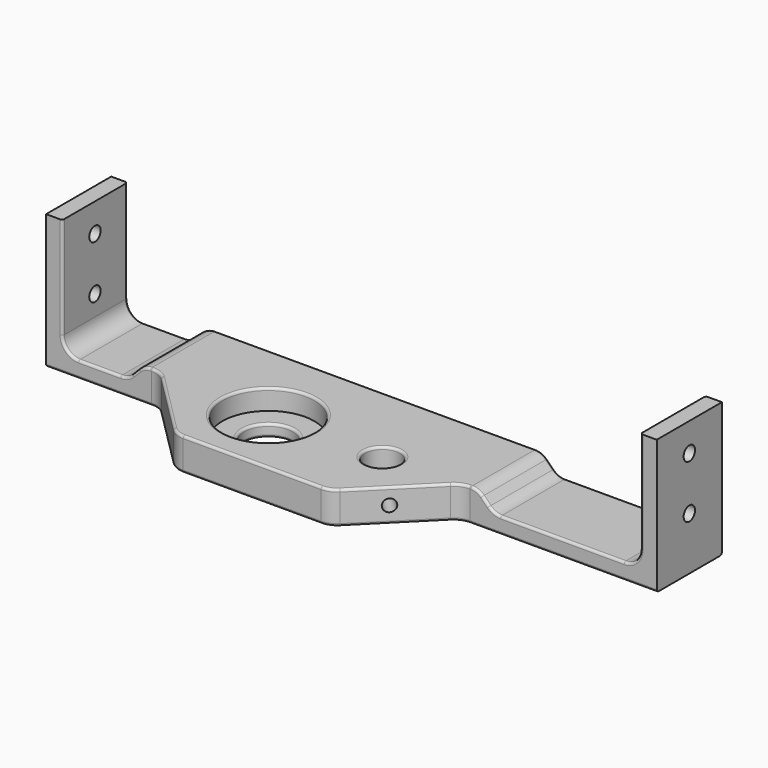
from build123d import *

# Parameters (mm, degrees)
F0_R      = 11.3
F0_R_2    = 4.3
F1_DEPTH  = 8
F0_R_3    = 6
F2_DEPTH  = 3
F4_W      = 4
F4_H      = 20
F5_DEPTH  = 25
F7_DEPTH  = 25
F8_R      = 0.6
F9_R      = 5
F10_R     = 4
F11_R     = 1.75
F12_DEPTH = 150.001
F13_R     = 0.6
F14_R     = 1.5
F15_DEPTH = 15


with BuildPart() as f1:
    # F0 (on Top) → F1 (new body)
    with BuildSketch(Plane.XY):
        Polygon((72.1656017255, 12.1974679563), (-77.8343982745, 12.1974679563), (-77.8343982745, -7.8025320437), (-49.8343982745, -7.8025320437), (-31.8343982745, -25.8025320437), (6.1656017255, -25.8025320437), (24.1656017255, -7.8025320437), (72.1656017255, -7.8025320437), align=None)
        with Locations((-22.4343982745, -8.8025320437)):
            Circle(F0_R, mode=Mode.SUBTRACT)
        with Locations((5.5656017255, -8.8025320437)):
            Circle(F0_R_2, mode=Mode.SUBTRACT)
    extrude(amount=F1_DEPTH)

    # F0 (on Top) → F2 (join)
    with BuildSketch(Plane.XY):
        with Locations((-22.4343982745, -8.8025320437)):
            Circle(F0_R)
        with Locations((-22.4343982745, -8.8025320437)):
            Circle(F0_R_3, mode=Mode.SUBTRACT)
    extrude(amount=F2_DEPTH)

    # F4 (on face) → F5 (join)
    with BuildSketch(Plane.XY.offset(8)):
        with Locations((70.1656017255, 2.1974679563)):
            Rectangle(F4_W, F4_H)
        with Locations((-75.8343982745, 2.1974679563)):
            Rectangle(F4_W, F4_H)
    extrude(amount=F5_DEPTH)

    # F6 (on face) → F7 (cut)
    with BuildSketch(Plane(origin=(0, 12.1974679563, 0), x_dir=(-1, 0, 0), z_dir=(0, 1, 0))):
        Polygon((-28.1656017255, 8), (-68.1656017255, 8), (-68.1656017255, 4), (-32.1656017255, 4), align=None)
        Polygon((73.8343982745, 8), (53.8343982745, 8), (57.8343982745, 4), (73.8343982745, 4), align=None)
    extrude(amount=-F7_DEPTH, mode=Mode.SUBTRACT)

    # F8
    f8_edges = [f1.edges().sort_by_distance(p)[0] for p in [
        (-28.434398, -8.802532, 0),
        (1.265602, -8.802532, 0),
        (-33.734398, -8.802532, 8),
        (-28.434398, -8.802532, 3),
        (1.265602, -8.802532, 8),
    ]]
    fillet(f8_edges, radius=F8_R)

    # F9
    f9_edges = [f1.edges().sort_by_distance(p)[0] for p in [
        (-49.834398, -7.802532, 4),
        (-31.834398, -25.802532, 4),
        (6.165602, -25.802532, 4),
        (24.165602, -7.802532, 4),
    ]]
    fillet(f9_edges, radius=F9_R)

    # F10
    f10_edges = [f1.edges().sort_by_distance(p)[0] for p in [
        (68.165602, 2.197468, 4),
        (-73.834398, 2.197468, 4),
        (32.165602, 2.197468, 4),
        (28.165602, 2.197468, 8),
        (-53.834398, 2.197468, 8),
        (-57.834398, 2.197468, 4),
    ]]
    fillet(f10_edges, radius=F10_R)

    # F11 (on face) → F12 (cut, through all)
    with BuildSketch(Plane.YZ.offset(72.1656017255)):
        with Locations((2.1974679563, 26)):
            Circle(F11_R)
        with Locations((2.1974679563, 13)):
            Circle(F11_R)
    extrude(amount=-F12_DEPTH, mode=Mode.SUBTRACT)

    # F13
    f13_edges = [f1.edges().sort_by_distance(p)[0] for p in [
        (-49.992049, -8.183134, 0),
        (-12.834398, 12.197468, 8),
        (-2.834398, 12.197468, 0),
        (-52.041505, -7.802532, 8),
        (-49.992049, -8.183134, 8),
        (-40.834398, -16.802532, 8),
        (-31.676748, -25.42193, 8),
        (26.372709, -7.802532, 8),
        (-12.834398, -25.802532, 8),
        (24.323252, -8.183134, 8),
        (6.007951, -25.42193, 8),
        (15.165602, -16.802532, 8),
        (-53.708278, -7.802532, 7.695518),
        (-55.834398, -7.802532, 6),
        (-64.869932, -7.802532, 0),
        (-57.960519, -7.802532, 4.304482),
        (-64.662825, -7.802532, 4),
        (-72.662825, -7.802532, 5.171573),
        (-73.834398, -7.802532, 20.5),
        (-53.708278, 12.197468, 7.695518),
        (68.165602, 12.197468, 20.5),
        (66.994029, 12.197468, 5.171573),
        (48.994029, 12.197468, 4),
        (32.291722, 12.197468, 4.304482),
        (30.165602, 12.197468, 6),
        (28.039481, 12.197468, 7.695518),
        (-73.834398, 12.197468, 20.5),
        (-72.662825, 12.197468, 5.171573),
        (-55.834398, 12.197468, 6),
        (-64.662825, 12.197468, 4),
        (-57.960519, 12.197468, 4.304482),
        (-40.834398, -16.802532, 0),
        (28.039481, -7.802532, 7.695518),
        (-31.676748, -25.42193, 0),
        (30.165602, -7.802532, 6),
        (49.201136, -7.802532, 0),
        (32.291722, -7.802532, 4.304482),
        (48.994029, -7.802532, 4),
        (66.994029, -7.802532, 5.171573),
        (68.165602, -7.802532, 20.5),
        (-12.834398, -25.802532, 0),
        (24.323252, -8.183134, 0),
        (6.007951, -25.42193, 0),
        (15.165602, -16.802532, 0),
    ]]
    fillet(f13_edges, radius=F13_R)

    # F14 (on face) → F15 (cut)
    with BuildSketch(Plane(origin=(15.9840668846, -15.9840668846, 0), x_dir=(0.7071067812, 0.7071067812, 0), z_dir=(0.7071067812, -0.7071067812, 0))):
        with Locations((-2.2962181829, 4)):
            Circle(F14_R)
    extrude(amount=-F15_DEPTH, mode=Mode.SUBTRACT)


solid = f1.part
